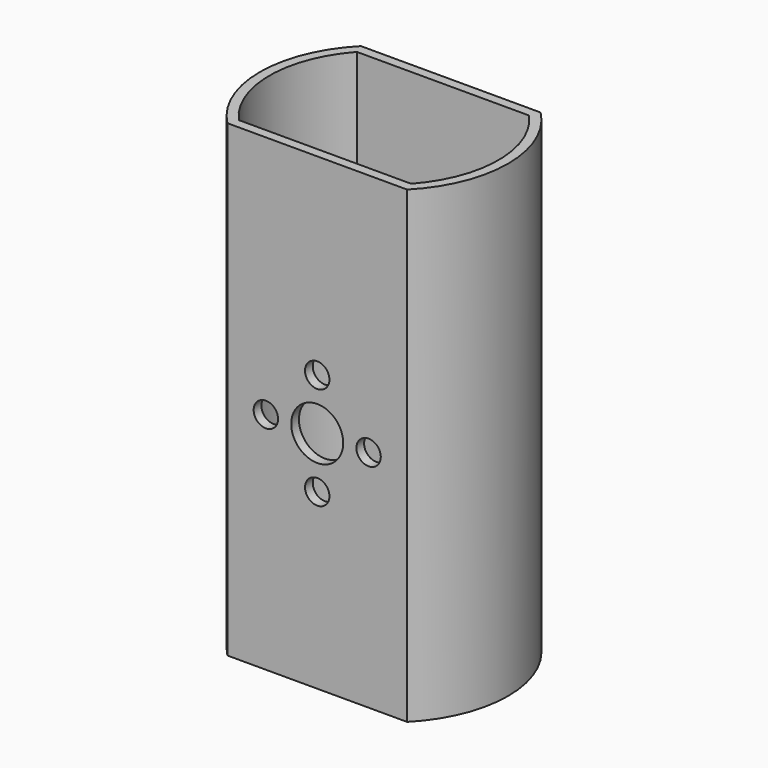
from build123d import *

# Parameters (mm, degrees)
F1_DEPTH = 3
F3_DEPTH = 70
F4_R     = 1.9
F4_R_2   = 4.05
F5_DEPTH = 4


# Not quite as in the source:
# - a feature names something its author has since deleted; it is built from what else it names


with BuildPart() as f1:
    # F0 (on Top) → F1 (new body)
    with BuildSketch(Plane.XY):
        with BuildLine():
            Line((14, 13), (-14, 13))
            ThreePointArc((-14, 13), (-19.3340623478, 0), (-14, -13))
            Line((-14, -13), (14, -13))
            ThreePointArc((14, -13), (19.3340623478, 0), (14, 13))
        make_face()
    extrude(amount=F1_DEPTH)

    # F2 (on face) → F3 (join)
    with BuildSketch(Plane.XY.offset(3)):
        with BuildLine():
            ThreePointArc((14, -13), (19.3340623478, 0), (14, 13))
            Line((14, 13), (-14, 13))
            ThreePointArc((-14, 13), (-19.3340623478, 0), (-14, -13))
            Line((-14, -13), (14, -13))
        make_face()
        with BuildLine():
            Line((13.4202267877, -11.5), (-13.4202267877, -11.5))
            ThreePointArc((-13.4202267877, -11.5), (-17.8340623478, 0), (-13.4202267877, 11.5))
            Line((-13.4202267877, 11.5), (13.4202267877, 11.5))
            ThreePointArc((13.4202267877, 11.5), (17.8340623478, 0), (13.4202267877, -11.5))
        make_face(mode=Mode.SUBTRACT)
    extrude(amount=F3_DEPTH)

    # F4 (on face) → F5 (cut)
    with BuildSketch(Plane.XZ.offset(13)):
        with Locations((-8, 35)):
            Circle(F4_R)
        with Locations((0, 35)):
            Circle(F4_R_2)
        with Locations((8, 35)):
            Circle(F4_R)
        with Locations((0, 43)):
            Circle(F4_R)
        with Locations((0, 27)):
            Circle(F4_R)
    extrude(amount=-F5_DEPTH, mode=Mode.SUBTRACT)


solid = f1.part
